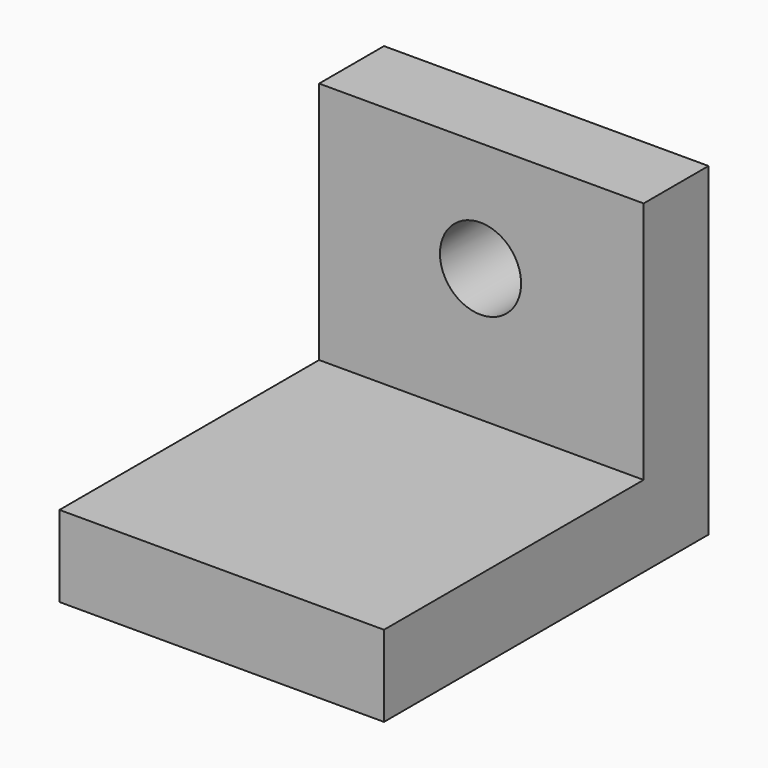
from build123d import *

# Parameters (mm, degrees)
F0_W     = 50.8
F0_H     = 50.8
F1_DEPTH = 12.7
F2_W     = 50.8
F2_H     = 50.8
F3_DEPTH = 12.7
F6_D     = 12.7


with BuildPart() as f1:
    # F0 (on Front) → F1 (new body)
    with BuildSketch(Plane.XZ):
        with Locations((-2.4638399482, 11.9818727014)):
            Rectangle(F0_W, F0_H)
    extrude(amount=F1_DEPTH)

    # F2 (on face) → F3 (join)
    with BuildSketch(Plane(origin=(0, 0, -13.4181272986), x_dir=(1, 0, 0), z_dir=(0, 0, -1))):
        with Locations((-2.4638399482, 38.1)):
            Rectangle(F2_W, F2_H)
    extrude(amount=-F3_DEPTH)

    # F6 (through all)
    with Locations(Plane.XZ.offset(12.7)):
        with Locations((-2.5935145095, 20.0997553766)):
            Hole(F6_D / 2)


solid = f1.part
